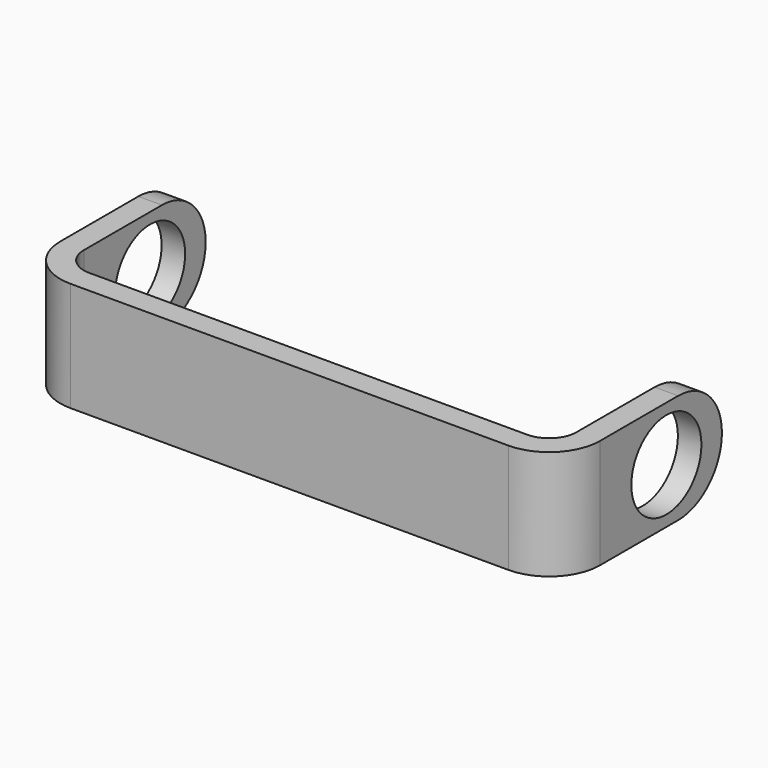
from build123d import *

# Parameters (mm, degrees)
F1_DEPTH = 2.54
F2_R     = 2.53999
F4_D     = 4.064
F4_DEPTH = 12.5231992362
F5_D     = 4.064


# Not quite as in the source:
# - a fillet or chamfer is up to 0.001 mm smaller than in the source, because OpenCascade refuses the exact size


with BuildPart() as f1:
    # F0 (on Top) → F1 (new body, symmetric)
    with BuildSketch(Plane.XY):
        with BuildLine():
            Line((-12.5221992362, 9.4272772469), (-12.5221992362, 8.3157558613))
            Line((-12.5221992362, 8.3157558613), (-12.5221992362, 2.3621992362))
            ThreePointArc((-12.5221992362, 2.3621992362), (-11.8303270984, 0.6918721378), (-10.16, 0))
            Line((-10.16, 0), (0, 0))
            Line((0, 0), (10.16, 0))
            ThreePointArc((10.16, 0), (11.8303270984, 0.6918721378), (12.5221992362, 2.3621992362))
            Line((12.5221992362, 2.3621992362), (12.5221992362, 8.3157558613))
            Line((12.5221992362, 8.3157558613), (12.5221992362, 9.4272772469))
            Line((12.5221992362, 9.4272772469), (11.43, 9.4272772469))
            Line((11.43, 9.4272772469), (11.43, 8.3157558613))
            Line((11.43, 8.3157558613), (11.43, 2.3621992362))
            ThreePointArc((11.43, 2.3621992362), (11.0580256121, 1.464173624), (10.16, 1.0921992362))
            Line((10.16, 1.0921992362), (1.2192031136, 1.0921992362))
            Line((1.2192031136, 1.0921992362), (0, 1.0921992362))
            Line((0, 1.0921992362), (-10.16, 1.0921992362))
            ThreePointArc((-10.16, 1.0921992362), (-11.0580256121, 1.464173624), (-11.43, 2.3621992362))
            Line((-11.43, 2.3621992362), (-11.43, 8.3157558613))
            Line((-11.43, 8.3157558613), (-11.43, 9.4272772469))
            Line((-11.43, 9.4272772469), (-12.5221992362, 9.4272772469))
        make_face()
    extrude(amount=F1_DEPTH, both=True)

    # F2 (radius 2.54 in the source; OpenCascade refuses exactly that, so slightly less here)
    f2_edges = [f1.edges().sort_by_distance(p)[0] for p in [
        (-11.9761, 9.427277, 2.54),
        (-11.9761, 9.427277, -2.54),
        (11.9761, 9.427277, 2.54),
        (11.9761, 9.427277, -2.54),
    ]]
    fillet(f2_edges, radius=F2_R)

    # F4 (through all, one way)
    with BuildSketch(Plane(origin=(0, 0, 0), x_dir=(0, 1, 0), z_dir=(-1, 0, 0))):
        with Locations((6.2061757781, 0)):
            Circle(F4_D / 2)
    extrude(amount=-F4_DEPTH, mode=Mode.SUBTRACT)

    # F5 (through all)
    with Locations(Plane.YZ):
        with Locations((6.2061757781, 0)):
            Hole(F5_D / 2)


solid = f1.part
